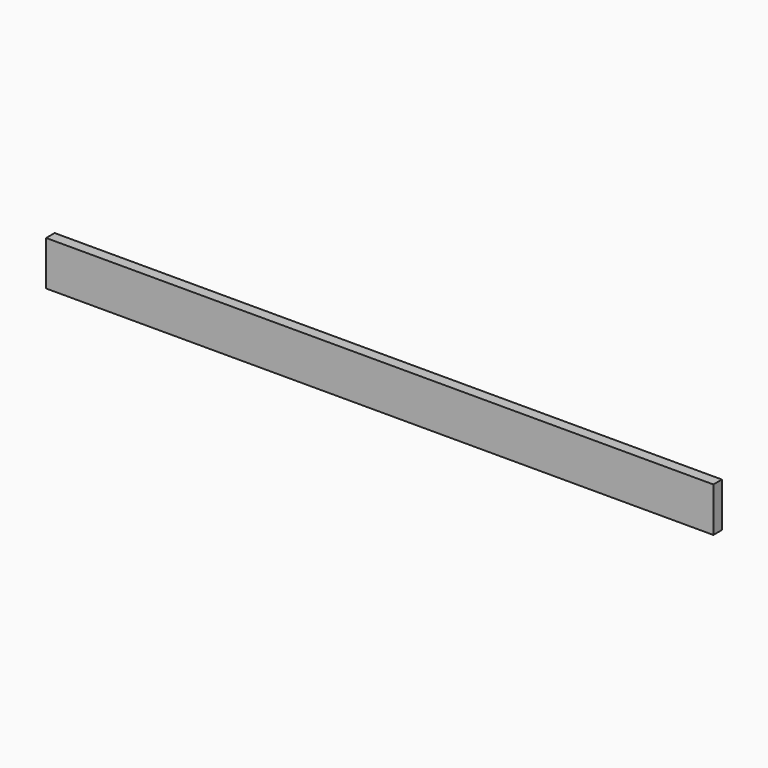
from build123d import *

# Parameters (mm, degrees)
F0_W     = 750
F0_H     = 50
F1_DEPTH = 12


# Not quite as in the source:
# - a feature names something its author has since deleted; it is built from what else it names


with BuildPart() as f1:
    # F0 (on Front) → F1 (new body)
    with BuildSketch(Plane.XZ):
        with Locations((375, 25)):
            Rectangle(F0_W, F0_H)
    extrude(amount=F1_DEPTH)


solid = f1.part
